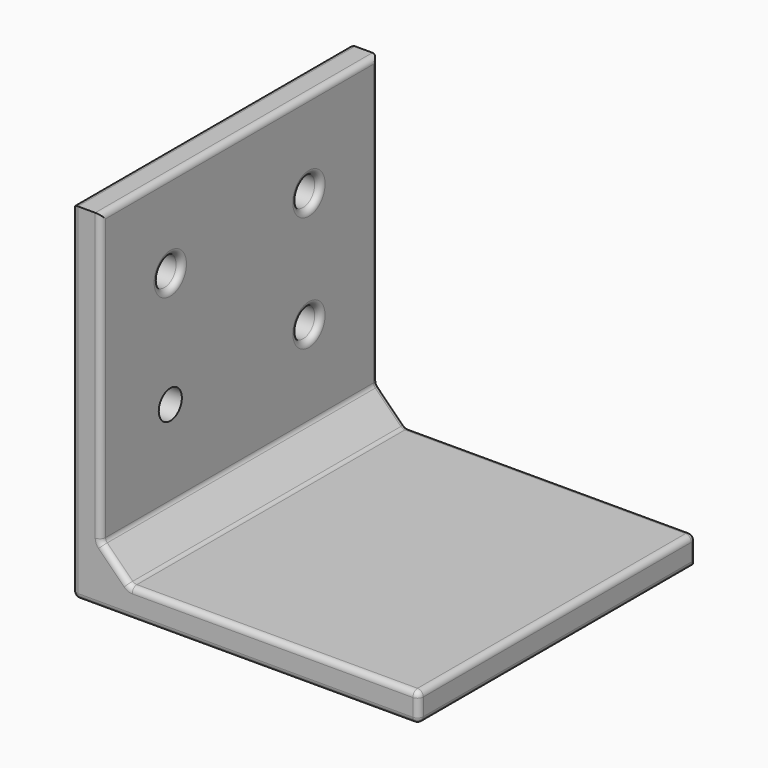
from build123d import *

# Parameters (mm, degrees)
F1_DEPTH = 76.2
F2_SIZE  = 6.35
F4_R     = 3.175
F5_DEPTH = 76.201
F6_F1_R  = 1.27
F6_F2_R  = 1.27


with BuildPart() as f1:
    # F0 (on Front) → F1 (new body)
    with BuildSketch(Plane.XZ):
        Polygon((0, 76.2), (0, 0), (76.2, 0), (76.2, 6.35), (6.35, 6.35), (6.35, 76.2), align=None)
    extrude(amount=F1_DEPTH)

    # F2
    f2_edges = [f1.edges().sort_by_distance(p)[0] for p in [
        (6.35, -38.1, 6.35),
    ]]
    chamfer(f2_edges, length=F2_SIZE)

    # F4 (on offset) → F5 (cut, through all)
    with BuildSketch(Plane(origin=(0, 0, 0), x_dir=(0, -1, 0), z_dir=(-1, 0, 0))):
        with Locations((19.05, 57.15)):
            Circle(F4_R)
        with Locations((19.05, 31.75)):
            Circle(F4_R)
        with Locations((57.15, 31.75)):
            Circle(F4_R)
        with Locations((57.15, 57.15)):
            Circle(F4_R)
    extrude(amount=-F5_DEPTH, mode=Mode.SUBTRACT)

    # F6: fillet of radius 1.27 on 23 edges, made by hand

    # F6_f1
    f6_f1_edges = [f1.edges().sort_by_distance(p)[0] for p in [
        (6.35, -38.1, 12.7),
        (12.7, -38.1, 6.35),
    ]]
    fillet(f6_f1_edges, radius=F6_F1_R)

    # F6_f2
    f6_f2_edges = [f1.edges().sort_by_distance(p)[0] for p in [
        (6.35, -53.975, 57.15),
        (6.35, -15.875, 57.15),
        (0, -53.975, 31.75),
        (6.35, -15.875, 31.75),
        (76.2, -38.1, 6.35),
        (44.7130256121, -76.2, 6.35),
        (44.7130256121, 0, 6.35),
        (6.35, 0, 44.7130256121),
        (6.35, -76.2, 44.7130256121),
        (6.35, -38.1, 76.2),
        (76.2, -38.1, 0),
        (76.2, -76.2, 3.175),
        (76.2, 0, 3.175),
        (38.1, -76.2, 0),
        (0, -76.2, 38.1),
        (0, -15.875, 57.15),
        (0, -53.975, 57.15),
        (0, -15.875, 31.75),
        (0, -38.1, 76.2),
        (0, 0, 38.1),
        (0, -38.1, 0),
        (6.4466729937, -76.2, 12.7400432651),
        (6.4466729937, 0, 12.7400432651),
        (12.7400432651, 0, 6.4466729937),
        (12.7400432651, -76.2, 6.4466729937),
    ]]
    fillet(f6_f2_edges, radius=F6_F2_R)


solid = f1.part
